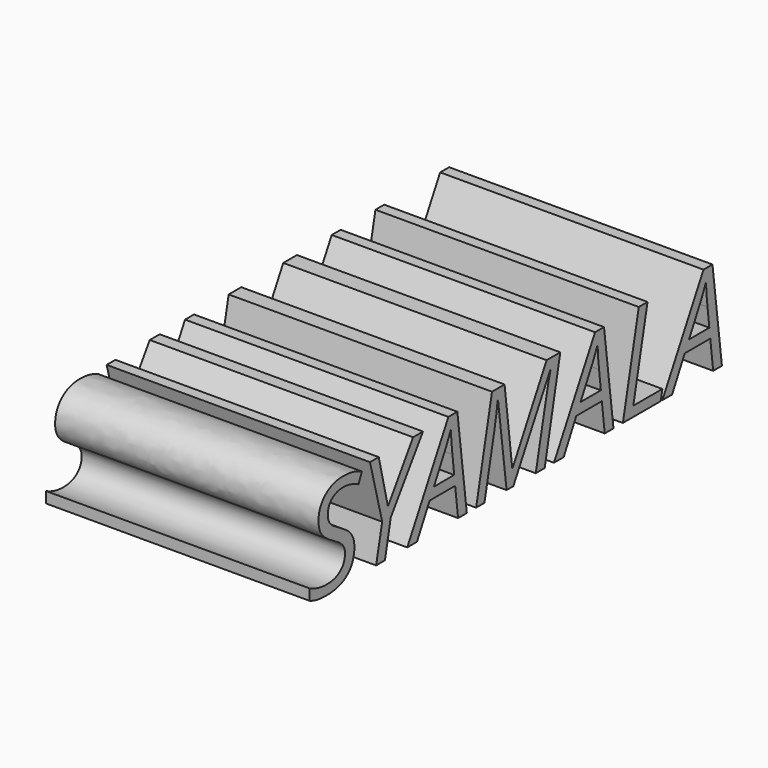
from build123d import *

# Parameters (mm, degrees)
F0_TEXT_SIZE = 12.5034189036
F1_DEPTH     = 25


# Not quite as in the source:
# - Text() gives the source's letters only with a copy of the font that has no kerning and outlines rounded to 1/6400 em; it was checked with that copy


with BuildPart() as f1:
    # F0 (on Right) → F1 (new body)
    with BuildSketch(Plane.YZ):
        with Locations((-27.5522676199, -6.396754865)):
            Text('SYAMALA', F0_TEXT_SIZE, font='Open Sans', font_style=FontStyle.ITALIC, text_align=(TextAlign.LEFT, TextAlign.BOTTOM))
    extrude(amount=F1_DEPTH)


solid = f1.part
